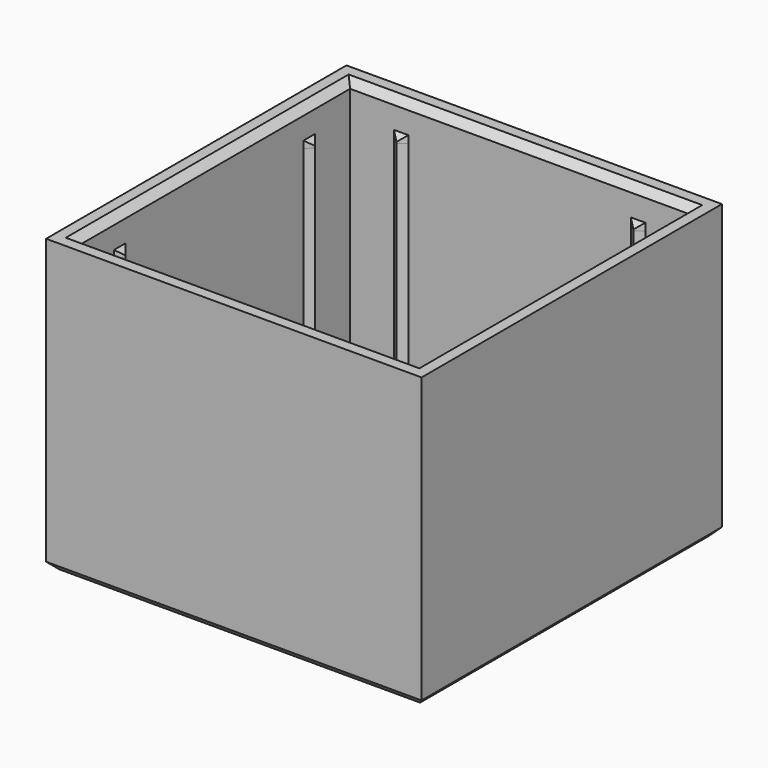
from build123d import *

# Parameters (mm, degrees)
F0_W          = 51.5
F0_H          = 51.5
F1_DEPTH      = 40
F2_DEPTH      = 35
F0_R          = 6
F3_DEPTH      = 2
F4_T4_DEPTH   = 7.1433659759
F4_T10_DEPTH  = 7.1433659759
F4_T16_DEPTH  = 7.1433659759
F4_T22_DEPTH  = 7.1433659759
F4_T28_DEPTH  = 7.1433659759
F4_T34_DEPTH  = 7.1433659759
F4_T40_DEPTH  = 7.1433659759
F4_T46_DEPTH  = 7.1433659759
F4_T49_DEPTH  = 46.5
F4_T51_DEPTH  = 46.5
F4_T53_DEPTH  = 56.6433659759
F4_T55_DEPTH  = 56.6433659759
F4_T63_DEPTH  = 49.071682988
F4_T67_DEPTH  = 49.071682988
F4_T74_DEPTH  = 49.071682988
F4_T78_DEPTH  = 49.071682988
F4_T85_DEPTH  = 49.071682988
F4_T89_DEPTH  = 49.071682988
F4_T96_DEPTH  = 49.071682988
F4_T100_DEPTH = 49.071682988


# Not quite as in the source:
# - a fillet or chamfer that OpenCascade refuses, or shapes differently, is made with other operations: its cross-section is extruded or revolved along the edge and cut away or added


with BuildPart() as f1:
    # F0 (on Top) → F1 (new body)
    with BuildSketch(Plane.XY):
        Rectangle(F0_W, F0_H)
        Polygon((-23.25, 17.25), (-23.25, 23.25), (-17.25, 23.25), (-15.25, 23.25), (15.25, 23.25), (17.25, 23.25), (23.25, 23.25), (23.25, 17.25), (23.25, 15.25), (23.25, -15.25), (23.25, -17.25), (23.25, -23.25), (17.25, -23.25), (15.25, -23.25), (-15.25, -23.25), (-17.25, -23.25), (-23.25, -23.25), (-23.25, -17.25), (-23.25, -15.25), (-23.25, 15.25), align=None, mode=Mode.SUBTRACT)
    extrude(amount=F1_DEPTH)

    # F0 (on Top) → F2 (join)
    with BuildSketch(Plane.XY):
        Rectangle(F0_W, F0_H)
        Polygon((-23.25, 17.25), (-23.25, 23.25), (-17.25, 23.25), (-15.25, 23.25), (15.25, 23.25), (17.25, 23.25), (23.25, 23.25), (23.25, 17.25), (23.25, 15.25), (23.25, -15.25), (23.25, -17.25), (23.25, -23.25), (17.25, -23.25), (15.25, -23.25), (-15.25, -23.25), (-17.25, -23.25), (-23.25, -23.25), (-23.25, -17.25), (-23.25, -15.25), (-23.25, 15.25), align=None, mode=Mode.SUBTRACT)
        Polygon((-22.45, 16.25), (-23.25, 17.25), (-23.25, 15.25), align=None)
        Polygon((-15.25, 23.25), (-17.25, 23.25), (-16.25, 22.45), align=None)
        Polygon((17.25, 23.25), (15.25, 23.25), (16.25, 22.45), align=None)
        Polygon((23.25, 15.25), (23.25, 17.25), (22.45, 16.25), align=None)
        Polygon((23.25, -17.25), (23.25, -15.25), (22.45, -16.25), align=None)
        Polygon((16.25, -22.45), (15.25, -23.25), (17.25, -23.25), align=None)
        Polygon((-16.25, -22.45), (-17.25, -23.25), (-15.25, -23.25), align=None)
        Polygon((-22.45, -16.25), (-23.25, -15.25), (-23.25, -17.25), align=None)
    extrude(amount=F2_DEPTH)

    # F0 (on Top) → F3 (join)
    with BuildSketch(Plane.XY):
        Polygon((-17.25, 23.25), (-23.25, 23.25), (-23.25, 17.25), (-22.45, 16.25), (-23.25, 15.25), (-23.25, -15.25), (-22.45, -16.25), (-23.25, -17.25), (-23.25, -23.25), (-17.25, -23.25), (-16.25, -22.45), (-15.25, -23.25), (15.25, -23.25), (16.25, -22.45), (17.25, -23.25), (23.25, -23.25), (23.25, -17.25), (22.45, -16.25), (23.25, -15.25), (23.25, 15.25), (22.45, 16.25), (23.25, 17.25), (23.25, 23.25), (17.25, 23.25), (16.25, 22.45), (15.25, 23.25), (-15.25, 23.25), (-16.25, 22.45), align=None)
        Circle(F0_R, mode=Mode.SUBTRACT)
    extrude(amount=F3_DEPTH)

    # F4: chamfer of 1 on 17 edges, made by hand


with BuildPart() as f4_tool2:
    # F4_s3 → F4_t4 (new body)
    with BuildSketch(Plane.YZ.offset(12.678317012)):
        Polygon((23.25, 36), (22.25, 35), (23.25, 35), align=None)
    extrude(amount=F4_T4_DEPTH)

    split(bisect_by=Plane(origin=(17.2926829268, 21.6158536585, 0), x_dir=(0, 0, 1), z_dir=(0.6246950476, 0.7808688094, 0)), keep=Keep.TOP)

    split(bisect_by=Plane(origin=(-4.6097560976, 5.762195122, 0), x_dir=(0, 0, 1), z_dir=(-0.6246950476, 0.7808688094, 0)), keep=Keep.TOP)


with BuildPart() as f1_1:
    add(f1.part)

    # F4_t1: union F4_tool2
    add(f4_tool2.part)


with BuildPart() as f4_tool8:
    # F4_s9 → F4_t10 (new body)
    with BuildSketch(Plane.YZ.offset(-19.821682988)):
        Polygon((23.25, 36), (22.25, 35), (23.25, 35), align=None)
    extrude(amount=F4_T10_DEPTH)

    split(bisect_by=Plane(origin=(4.6097560976, 5.762195122, 0), x_dir=(0, 0, 1), z_dir=(0.6246950476, 0.7808688094, 0)), keep=Keep.TOP)

    split(bisect_by=Plane(origin=(-17.2926829268, 21.6158536585, 0), x_dir=(0, 0, 1), z_dir=(-0.6246950476, 0.7808688094, 0)), keep=Keep.TOP)


with BuildPart() as f1_2:
    add(f1_1.part)

    # F4_t7: union F4_tool8
    add(f4_tool8.part)


with BuildPart() as f4_tool14:
    # F4_s15 → F4_t16 (new body)
    with BuildSketch(Plane.XZ.offset(12.678317012)):
        Polygon((23.25, 36), (22.25, 35), (23.25, 35), align=None)
    extrude(amount=F4_T16_DEPTH)

    split(bisect_by=Plane(origin=(21.6158536585, -17.2926829268, 0), x_dir=(0, 0, 1), z_dir=(0.7808688094, -0.6246950476, 0)), keep=Keep.TOP)

    split(bisect_by=Plane(origin=(5.762195122, 4.6097560976, 0), x_dir=(0, 0, 1), z_dir=(0.7808688094, 0.6246950476, 0)), keep=Keep.TOP)


with BuildPart() as f1_3:
    add(f1_2.part)

    # F4_t13: union F4_tool14
    add(f4_tool14.part)


with BuildPart() as f4_tool20:
    # F4_s21 → F4_t22 (new body)
    with BuildSketch(Plane.XZ.offset(-19.821682988)):
        Polygon((23.25, 36), (22.25, 35), (23.25, 35), align=None)
    extrude(amount=F4_T22_DEPTH)

    split(bisect_by=Plane(origin=(5.762195122, -4.6097560976, 0), x_dir=(0, 0, 1), z_dir=(0.7808688094, -0.6246950476, 0)), keep=Keep.TOP)

    split(bisect_by=Plane(origin=(21.6158536585, 17.2926829268, 0), x_dir=(0, 0, 1), z_dir=(0.7808688094, 0.6246950476, 0)), keep=Keep.TOP)


with BuildPart() as f1_4:
    add(f1_3.part)

    # F4_t19: union F4_tool20
    add(f4_tool20.part)


with BuildPart() as f4_tool26:
    # F4_s27 → F4_t28 (new body)
    with BuildSketch(Plane.XZ.offset(-12.678317012)):
        Polygon((-23.25, 36), (-22.25, 35), (-23.25, 35), align=None)
    extrude(amount=-F4_T28_DEPTH)

    split(bisect_by=Plane(origin=(-21.6158536585, 17.2926829268, 0), x_dir=(0, 0, 1), z_dir=(-0.7808688094, 0.6246950476, 0)), keep=Keep.TOP)

    split(bisect_by=Plane(origin=(-5.762195122, -4.6097560976, 0), x_dir=(0, 0, 1), z_dir=(-0.7808688094, -0.6246950476, 0)), keep=Keep.TOP)


with BuildPart() as f1_5:
    add(f1_4.part)

    # F4_t25: union F4_tool26
    add(f4_tool26.part)


with BuildPart() as f4_tool32:
    # F4_s33 → F4_t34 (new body)
    with BuildSketch(Plane.XZ.offset(19.821682988)):
        Polygon((-23.25, 36), (-22.25, 35), (-23.25, 35), align=None)
    extrude(amount=-F4_T34_DEPTH)

    split(bisect_by=Plane(origin=(-5.762195122, 4.6097560976, 0), x_dir=(0, 0, 1), z_dir=(-0.7808688094, 0.6246950476, 0)), keep=Keep.TOP)

    split(bisect_by=Plane(origin=(-21.6158536585, -17.2926829268, 0), x_dir=(0, 0, 1), z_dir=(-0.7808688094, -0.6246950476, 0)), keep=Keep.TOP)


with BuildPart() as f1_6:
    add(f1_5.part)

    # F4_t31: union F4_tool32
    add(f4_tool32.part)


with BuildPart() as f4_tool38:
    # F4_s39 → F4_t40 (new body)
    with BuildSketch(Plane.YZ.offset(-12.678317012)):
        Polygon((-23.25, 36), (-22.25, 35), (-23.25, 35), align=None)
    extrude(amount=-F4_T40_DEPTH)

    split(bisect_by=Plane(origin=(-17.2926829268, -21.6158536585, 0), x_dir=(0, 0, 1), z_dir=(-0.6246950476, -0.7808688094, 0)), keep=Keep.TOP)

    split(bisect_by=Plane(origin=(4.6097560976, -5.762195122, 0), x_dir=(0, 0, 1), z_dir=(0.6246950476, -0.7808688094, 0)), keep=Keep.TOP)


with BuildPart() as f1_7:
    add(f1_6.part)

    # F4_t37: union F4_tool38
    add(f4_tool38.part)


with BuildPart() as f4_tool44:
    # F4_s45 → F4_t46 (new body)
    with BuildSketch(Plane.YZ.offset(19.821682988)):
        Polygon((-23.25, 36), (-22.25, 35), (-23.25, 35), align=None)
    extrude(amount=-F4_T46_DEPTH)

    split(bisect_by=Plane(origin=(-4.6097560976, -5.762195122, 0), x_dir=(0, 0, 1), z_dir=(-0.6246950476, -0.7808688094, 0)), keep=Keep.TOP)

    split(bisect_by=Plane(origin=(17.2926829268, -21.6158536585, 0), x_dir=(0, 0, 1), z_dir=(0.6246950476, -0.7808688094, 0)), keep=Keep.TOP)


with BuildPart() as f1_8:
    add(f1_7.part)

    # F4_t43: union F4_tool44
    add(f4_tool44.part)

    # F4_s50 → F4_t49 (cut)
    with BuildSketch(Plane.YZ.offset(-23.25)):
        Polygon((24.25, 40), (23.25, 39), (23.25, 40), align=None)
        Polygon((-24.25, 40), (-23.25, 39), (-23.25, 40), align=None)
    extrude(amount=F4_T49_DEPTH, mode=Mode.SUBTRACT)

    # F4_s52 → F4_t51 (cut)
    with BuildSketch(Plane.XZ.offset(-23.25)):
        Polygon((-24.25, 40), (-23.25, 39), (-23.25, 40), align=None)
        Polygon((24.25, 40), (23.25, 39), (23.25, 40), align=None)
    extrude(amount=F4_T51_DEPTH, mode=Mode.SUBTRACT)

    # F4_s54 → F4_t53 (cut)
    with BuildSketch(Plane.YZ.offset(-28.321682988)):
        Polygon((25.75, 1), (24.75, 0), (25.75, 0), align=None)
        Polygon((-25.75, 1), (-24.75, 0), (-25.75, 0), align=None)
    extrude(amount=F4_T53_DEPTH, mode=Mode.SUBTRACT)

    # F4_s56 → F4_t55 (cut)
    with BuildSketch(Plane.XZ.offset(-28.321682988)):
        Polygon((-25.75, 1), (-24.75, 0), (-25.75, 0), align=None)
        Polygon((25.75, 1), (24.75, 0), (25.75, 0), align=None)
    extrude(amount=F4_T55_DEPTH, mode=Mode.SUBTRACT)

    # F4_s57 → F4_t58 (revolve, cut)
    with BuildSketch(Plane.XZ):
        Polygon((6, 1), (7, 0), (6, 0), align=None)
    revolve(axis=Axis((0, 0, 0), (0, 0, 1)), mode=Mode.SUBTRACT)


with BuildPart() as f4_tool61:
    # F4_s62 → F4_t63 (new body)
    with BuildSketch(Plane.YZ.offset(25.821682988)):
        Polygon((24.25, 40), (23.25, 39), (23.25, 40), align=None)
    extrude(amount=-F4_T63_DEPTH)

    split(bisect_by=Plane.YZ.offset(23.25), keep=Keep.TOP)


with BuildPart() as f4_tool65:
    # F4_s66 → F4_t67 (new body)
    with BuildSketch(Plane.XZ.offset(23.25)):
        Polygon((24.25, 40), (23.25, 39), (23.25, 40), align=None)
    extrude(amount=-F4_T67_DEPTH)

    split(bisect_by=Plane.XZ.offset(-23.25), keep=Keep.BOTTOM)


with BuildPart() as f4_tool61_1:
    add(f4_tool61.part)

    # F4_t69: intersect F4_tool65
    add(f4_tool65.part, mode=Mode.INTERSECT)


with BuildPart() as f1_9:
    add(f1_8.part)

    # F4_t59: cut F4_tool61
    add(f4_tool61_1.part, mode=Mode.SUBTRACT)


with BuildPart() as f4_tool72:
    # F4_s73 → F4_t74 (new body)
    with BuildSketch(Plane.XZ.offset(-25.821682988)):
        Polygon((-24.25, 40), (-23.25, 39), (-23.25, 40), align=None)
    extrude(amount=F4_T74_DEPTH)

    split(bisect_by=Plane.XZ.offset(-23.25), keep=Keep.BOTTOM)


with BuildPart() as f4_tool76:
    # F4_s77 → F4_t78 (new body)
    with BuildSketch(Plane.YZ.offset(23.25)):
        Polygon((24.25, 40), (23.25, 39), (23.25, 40), align=None)
    extrude(amount=-F4_T78_DEPTH)

    split(bisect_by=Plane.YZ.offset(-23.25), keep=Keep.BOTTOM)


with BuildPart() as f4_tool72_1:
    add(f4_tool72.part)

    # F4_t80: intersect F4_tool76
    add(f4_tool76.part, mode=Mode.INTERSECT)


with BuildPart() as f1_10:
    add(f1_9.part)

    # F4_t70: cut F4_tool72
    add(f4_tool72_1.part, mode=Mode.SUBTRACT)


with BuildPart() as f4_tool83:
    # F4_s84 → F4_t85 (new body)
    with BuildSketch(Plane.XZ.offset(-23.25)):
        Polygon((-24.25, 40), (-23.25, 39), (-23.25, 40), align=None)
    extrude(amount=F4_T85_DEPTH)

    split(bisect_by=Plane.XZ.offset(23.25), keep=Keep.TOP)


with BuildPart() as f4_tool87:
    # F4_s88 → F4_t89 (new body)
    with BuildSketch(Plane.YZ.offset(-25.821682988)):
        Polygon((-24.25, 40), (-23.25, 39), (-23.25, 40), align=None)
    extrude(amount=F4_T89_DEPTH)

    split(bisect_by=Plane.YZ.offset(-23.25), keep=Keep.BOTTOM)


with BuildPart() as f4_tool83_1:
    add(f4_tool83.part)

    # F4_t91: intersect F4_tool87
    add(f4_tool87.part, mode=Mode.INTERSECT)


with BuildPart() as f1_11:
    add(f1_10.part)

    # F4_t81: cut F4_tool83
    add(f4_tool83_1.part, mode=Mode.SUBTRACT)


with BuildPart() as f4_tool94:
    # F4_s95 → F4_t96 (new body)
    with BuildSketch(Plane.XZ.offset(25.821682988)):
        Polygon((24.25, 40), (23.25, 39), (23.25, 40), align=None)
    extrude(amount=-F4_T96_DEPTH)

    split(bisect_by=Plane.XZ.offset(23.25), keep=Keep.TOP)


with BuildPart() as f4_tool98:
    # F4_s99 → F4_t100 (new body)
    with BuildSketch(Plane.YZ.offset(-23.25)):
        Polygon((-24.25, 40), (-23.25, 39), (-23.25, 40), align=None)
    extrude(amount=F4_T100_DEPTH)

    split(bisect_by=Plane.YZ.offset(23.25), keep=Keep.TOP)


with BuildPart() as f4_tool94_1:
    add(f4_tool94.part)

    # F4_t102: intersect F4_tool98
    add(f4_tool98.part, mode=Mode.INTERSECT)


with BuildPart() as f1_12:
    add(f1_11.part)

    # F4_t92: cut F4_tool94
    add(f4_tool94_1.part, mode=Mode.SUBTRACT)


solid = f1_12.part
